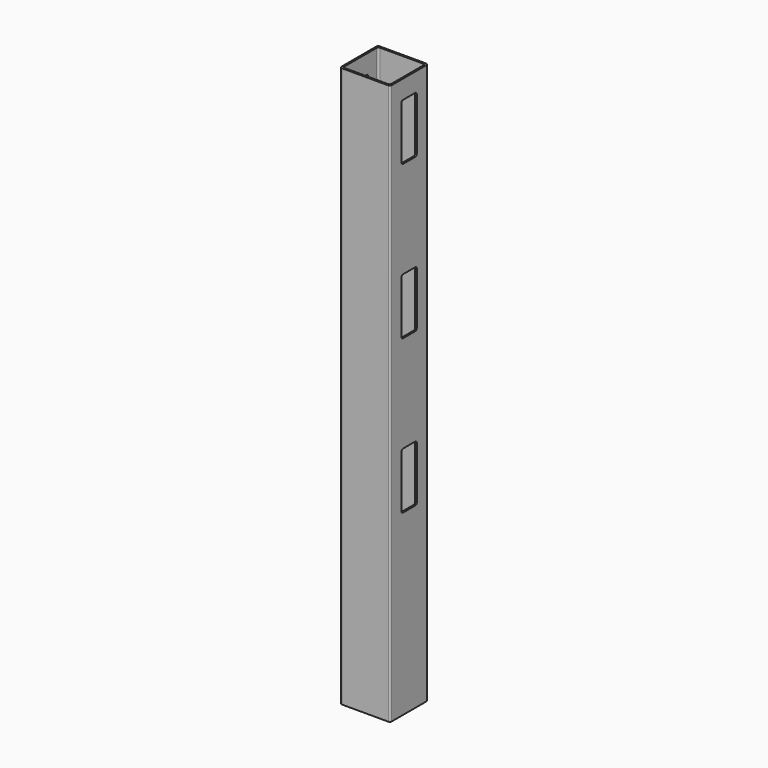
from build123d import *

# Parameters (mm, degrees)
F1_DEPTH = 1500
F4_DEPTH = 150


# Not quite as in the source:
# - the program builds the solid bodies; features that only make, move or delete a surface that nothing else refers to are left out


with BuildPart() as f1:
    # F0 (on Top) → F1 (new body)
    with BuildSketch(Plane.XY):
        with BuildLine():
            Line((-62.3253015232, -63.5), (62.3253015232, -63.5))
            ThreePointArc((62.3253015232, -63.5), (65.8608354292, -62.0355339059), (67.3253015232, -58.5))
            Line((67.3253015232, -58.5), (67.3253015232, 58.5))
            ThreePointArc((67.3253015232, 58.5), (65.8608354292, 62.0355339059), (62.3253015232, 63.5))
            Line((62.3253015232, 63.5), (-62.3253015232, 63.5))
            ThreePointArc((-62.3253015232, 63.5), (-65.8608354292, 62.0355339059), (-67.3253015232, 58.5))
            Line((-67.3253015232, 58.5), (-67.3253015232, -58.5))
            ThreePointArc((-67.3253015232, -58.5), (-65.8608354292, -62.0355339059), (-62.3253015232, -63.5))
        make_face()
        with BuildLine():
            Line((-57.8253015232, 59), (57.8253015232, 59))
            ThreePointArc((57.8253015232, 59), (61.3608354292, 57.5355339059), (62.8253015232, 54))
            Line((62.8253015232, 54), (62.8253015232, -54))
            ThreePointArc((62.8253015232, -54), (61.3608354292, -57.5355339059), (57.8253015232, -59))
            Line((57.8253015232, -59), (-57.8253015232, -59))
            ThreePointArc((-57.8253015232, -59), (-61.3608354292, -57.5355339059), (-62.8253015232, -54))
            Line((-62.8253015232, -54), (-62.8253015232, 54))
            ThreePointArc((-62.8253015232, 54), (-61.3608354292, 57.5355339059), (-57.8253015232, 59))
        make_face(mode=Mode.SUBTRACT)
    extrude(amount=F1_DEPTH)

    # F2 (on face) → F4 (cut)
    with BuildSketch(Plane.YZ.offset(67.3253015232)):
        with BuildLine():
            ThreePointArc((-25.5, 1304), (-24.0355339059, 1300.4644660941), (-20.5, 1299))
            Line((-20.5, 1299), (20.5, 1299))
            ThreePointArc((20.5, 1299), (24.0355339059, 1300.4644660941), (25.5, 1304))
            Line((25.5, 1304), (25.5, 1445))
            ThreePointArc((25.5, 1445), (24.0355339059, 1448.5355339059), (20.5, 1450))
            Line((20.5, 1450), (-20.5, 1450))
            ThreePointArc((-20.5, 1450), (-24.0355339059, 1448.5355339059), (-25.5, 1445))
            Line((-25.5, 1445), (-25.5, 1304))
        make_face()
        with BuildLine():
            ThreePointArc((-25.5, 893), (-24.0355339059, 889.4644660941), (-20.5, 888))
            Line((-20.5, 888), (20.5, 888))
            ThreePointArc((20.5, 888), (24.0355339059, 889.4644660941), (25.5, 893))
            Line((25.5, 893), (25.5, 1034))
            ThreePointArc((25.5, 1034), (24.0355339059, 1037.5355339059), (20.5, 1039))
            Line((20.5, 1039), (-20.5, 1039))
            ThreePointArc((-20.5, 1039), (-24.0355339059, 1037.5355339059), (-25.5, 1034))
            Line((-25.5, 1034), (-25.5, 893))
        make_face()
        with BuildLine():
            ThreePointArc((-25.5, 482), (-24.0355339059, 478.4644660941), (-20.5, 477))
            Line((-20.5, 477), (20.5, 477))
            ThreePointArc((20.5, 477), (24.0355339059, 478.4644660941), (25.5, 482))
            Line((25.5, 482), (25.5, 623))
            ThreePointArc((25.5, 623), (24.0355339059, 626.5355339059), (20.5, 628))
            Line((20.5, 628), (-20.5, 628))
            ThreePointArc((-20.5, 628), (-24.0355339059, 626.5355339059), (-25.5, 623))
            Line((-25.5, 623), (-25.5, 482))
        make_face()
    extrude(amount=-F4_DEPTH, mode=Mode.SUBTRACT)


solid = f1.part
